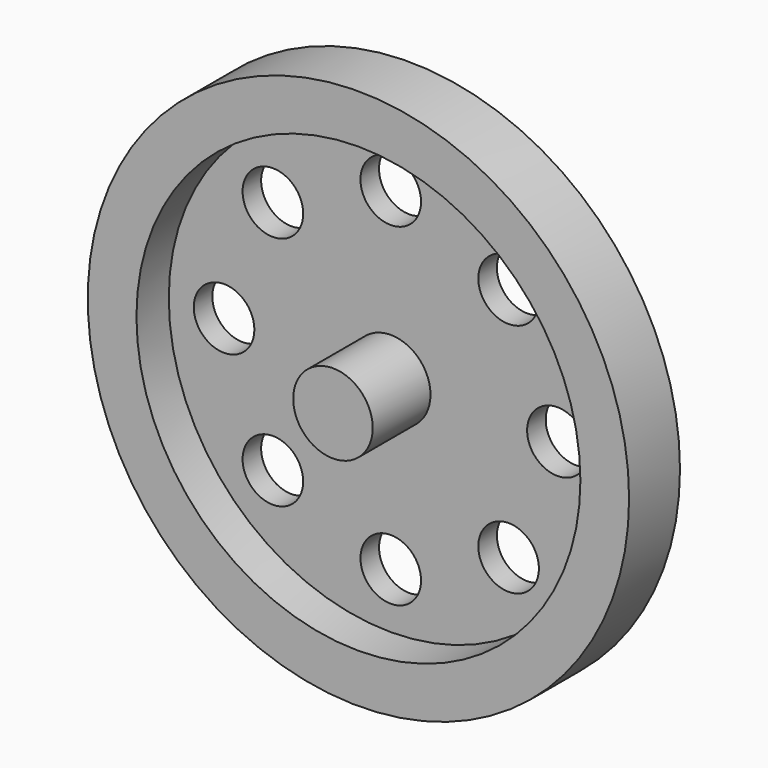
from build123d import *

# Parameters (mm, degrees)
F0_R      = 17.018
F1_DEPTH  = 4
F4_R      = 2.5
F5_DEPTH  = 2
F7_R      = 1.905
F8_DEPTH  = 25.4
F9_R      = 13.9564544628
F9_R_2    = 1.905
F9_R_3    = 2.5
F10_DEPTH = 2.54


# Not quite as in the source:
# - the program builds the solid bodies; features that only make, move or delete a surface that nothing else refers to are left out


with BuildPart() as f1:
    # F0 (on Front) → F1 (new body)
    with BuildSketch(Plane.XZ):
        Circle(F0_R)
    extrude(amount=-F1_DEPTH)

    # F4 (on Front) → F5 (join)
    with BuildSketch(Plane.XZ):
        Circle(F4_R)
    extrude(amount=F5_DEPTH)

    # F7 (on face) → F8 (cut)
    with BuildSketch(Plane.XZ):
        with Locations((-7.4105341768, 7.4105341768)):
            Circle(F7_R)
        with Locations((0, 10.4800779372)):
            Circle(F7_R)
        with Locations((7.4105341768, 7.4105341768)):
            Circle(F7_R)
        with Locations((10.4800779372, 0)):
            Circle(F7_R)
        with Locations((7.4105341768, -7.4105341768)):
            Circle(F7_R)
        with Locations((0, -10.4800779372)):
            Circle(F7_R)
        with Locations((-7.4105341768, -7.4105341768)):
            Circle(F7_R)
        with Locations((-10.4800779372, 0)):
            Circle(F7_R)
    extrude(amount=-F8_DEPTH, mode=Mode.SUBTRACT)

    # F9 (on face) → F10 (cut)
    with BuildSketch(Plane.XZ):
        Circle(F9_R)
        with Locations((-7.4105341768, -7.4105341768)):
            Circle(F9_R_2, mode=Mode.SUBTRACT)
        with Locations((0, -10.4800779372)):
            Circle(F9_R_2, mode=Mode.SUBTRACT)
        with Locations((7.4105341768, -7.4105341768)):
            Circle(F9_R_2, mode=Mode.SUBTRACT)
        with Locations((-10.4800779372, 0)):
            Circle(F9_R_2, mode=Mode.SUBTRACT)
        with Locations((-7.4105341768, 7.4105341768)):
            Circle(F9_R_2, mode=Mode.SUBTRACT)
        Circle(F9_R_3, mode=Mode.SUBTRACT)
        with Locations((7.4105341768, 7.4105341768)):
            Circle(F9_R_2, mode=Mode.SUBTRACT)
        with Locations((10.4800779372, 0)):
            Circle(F9_R_2, mode=Mode.SUBTRACT)
        with Locations((0, 10.4800779372)):
            Circle(F9_R_2, mode=Mode.SUBTRACT)
    extrude(amount=-F10_DEPTH, mode=Mode.SUBTRACT)


solid = f1.part
